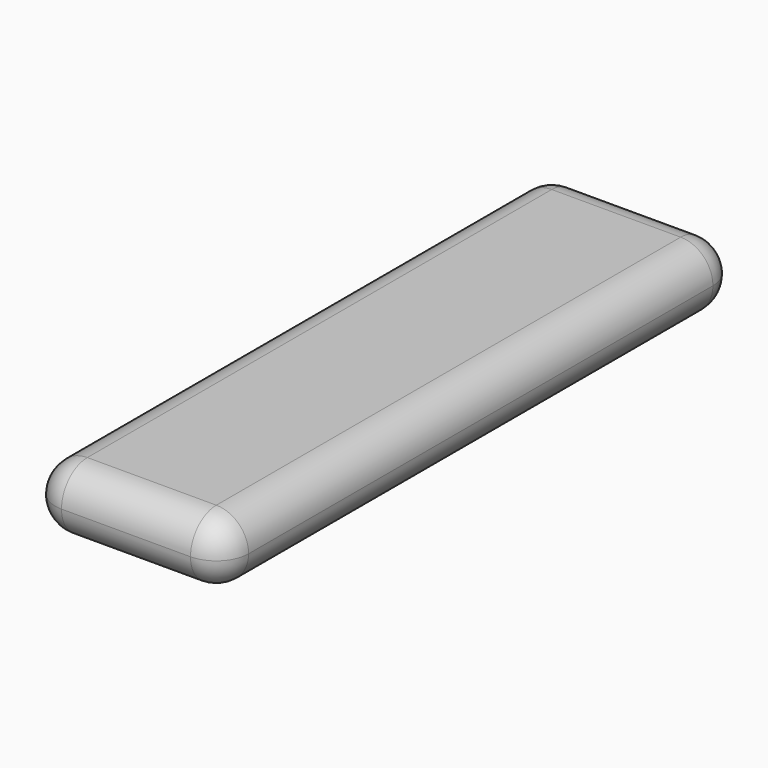
from build123d import *

# Parameters (mm, degrees)
F0_W     = 38.1
F0_H     = 127
F1_DEPTH = 12.7
F2_R     = 6.34999


# Not quite as in the source:
# - a fillet or chamfer is up to 0.001 mm smaller than in the source, because OpenCascade refuses the exact size


with BuildPart() as f1:
    # F0 (on Top) → F1 (new body)
    with BuildSketch(Plane.XY):
        Rectangle(F0_W, F0_H)
    extrude(amount=F1_DEPTH)

    # F2 (radius 6.35 in the source; OpenCascade refuses exactly that, so slightly less here)
    f2_edges = [f1.edges().sort_by_distance(p)[0] for p in [
        (-19.05, 0, 12.7),
        (-19.05, 0, 0),
        (19.05, 0, 0),
        (19.05, 0, 12.7),
        (0, -63.5, 0),
        (-19.05, -63.5, 6.35),
        (19.05, -63.5, 6.35),
        (0, -63.5, 12.7),
        (19.05, 63.5, 6.35),
        (-19.05, 63.5, 6.35),
        (0, 63.5, 0),
        (0, 63.5, 12.7),
    ]]
    fillet(f2_edges, radius=F2_R)


solid = f1.part
